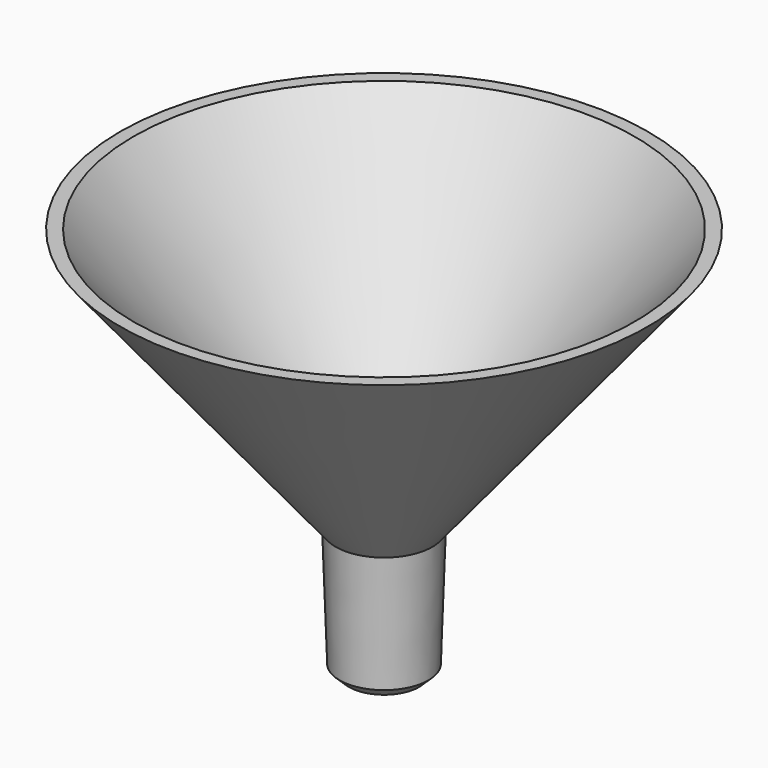
from build123d import *


# Not quite as in the source:
# - a fillet or chamfer that OpenCascade refuses, or shapes differently, is made with other operations: its cross-section is extruded or revolved along the edge and cut away or added


with BuildPart() as f2:
    # F0 (on Front) → F2 (revolve)
    with BuildSketch(Plane.XZ):
        Polygon((-10, -50.2272490659), (-8, -50.2272490659), (-8, -20.2272490659), (-56.9863888878, 39.7727509341), (-60, 39.7727509341), (-11, -20.2439203648), align=None)
    revolve(axis=Axis((0, 0, -35.9380319715), (0, 0, -1)))

    # F3: chamfer of 3 on 1 edges, made by hand

    # F3_s1 → F3_t2 (revolve, cut)
    with BuildSketch(Plane.XZ):
        Polygon((-10.1, -47.2289161958), (-7, -50.2272490659), (-10, -50.2272490659), align=None)
    revolve(axis=Axis((0, 0, -50.2272490659), (0, 0, -1)), mode=Mode.SUBTRACT)


solid = f2.part
